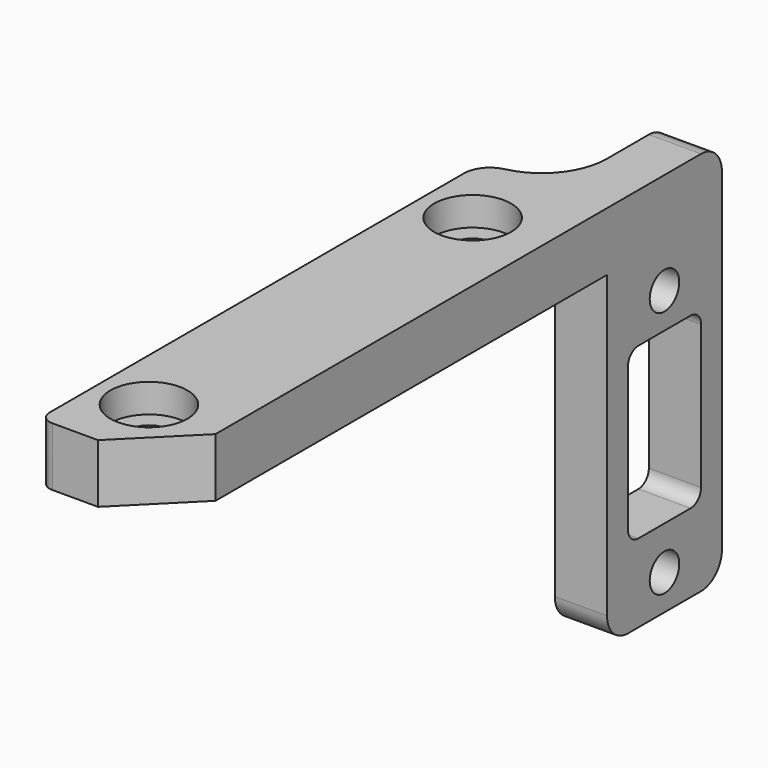
from build123d import *

# Parameters (mm, degrees)
F0_W           = 9.5
F0_H           = 42.5
F1_DEPTH       = 4.5
F3_D           = 3.1
F3_CBORE_D     = 5.9
F3_CBORE_DEPTH = 2.2
F4_W           = 11
F4_H           = 29.5
F5_DEPTH       = 4
F7_D           = 2.83
F8_W           = 7
F8_H           = 13
F9_DEPTH       = 25
F10_T1_DEPTH   = 4.5
F11_R          = 2
F12_SIZE       = 5
F13_R          = 1


# Not quite as in the source:
# - a fillet or chamfer that OpenCascade refuses, or shapes differently, is made with other operations: its cross-section is extruded or revolved along the edge and cut away or added


with BuildPart() as f1:
    # F0 (on Top) → F1 (new body)
    with BuildSketch(Plane.XY):
        with Locations((-4.75, 21.25)):
            Rectangle(F0_W, F0_H)
    extrude(amount=F1_DEPTH)

    # F3 (through all)
    with Locations(Plane.XY.offset(4.5)):
        with Locations((-5.5, 36.5), (-5.5, 5.5)):
            CounterBoreHole(F3_D / 2, F3_CBORE_D / 2, F3_CBORE_DEPTH)

    # F4 (on Right) → F5 (join)
    with BuildSketch(Plane.YZ):
        with Locations((48, -10.25)):
            Rectangle(F4_W, F4_H)
    extrude(amount=-F5_DEPTH)

    # F7 (through all)
    with Locations(Plane.YZ):
        with Locations((48, -3.3), (48, -22.3)):
            Hole(F7_D / 2)

    # F8 (on face) → F9 (cut)
    with BuildSketch(Plane.YZ):
        with Locations((48, -12.5)):
            Rectangle(F8_W, F8_H)
    extrude(amount=-F9_DEPTH, mode=Mode.SUBTRACT)

    # F10: fillet of radius 5 on 1 edges, made by hand

    # F10_s2 → F10_t1 (join)
    with BuildSketch(Plane.XY):
        with BuildLine():
            ThreePointArc((-9.0009656854, 42.4996), (-5.4644660941, 43.9644660941), (-3.9996, 47.5009656854))
            Line((-3.9996, 47.5009656854), (-3.4994634315, 47.5009656854))
            ThreePointArc((-3.4994634315, 47.5009656854), (-3.4998634315, 45.0004828427), (-3.4998634315, 42.5))
            Line((-3.4998634315, 42.5), (-4, 41.9998634315))
            ThreePointArc((-4, 41.9998634315), (-6.5004828427, 41.9998634315), (-9.0009656854, 41.9994634315))
            Line((-9.0009656854, 41.9994634315), (-9.0009656854, 42.4996))
        make_face()
    extrude(amount=F10_T1_DEPTH)

    # F11
    f11_edges = [f1.edges().sort_by_distance(p)[0] for p in [
        (-2, 53.5, 4.5),
        (-2, 53.5, -25),
        (-2, 42.5, -25),
        (-9.5, 42.5, 2.25),
    ]]
    fillet(f11_edges, radius=F11_R)

    # F12
    f12_edges = [f1.edges().sort_by_distance(p)[0] for p in [
        (0, 0, 2.25),
    ]]
    chamfer(f12_edges, length=F12_SIZE)

    # F13
    f13_edges = [f1.edges().sort_by_distance(p)[0] for p in [
        (-2, 44.5, -6),
        (-2, 51.5, -6),
        (-2, 44.5, -19),
        (-2, 51.5, -19),
        (-9.5, 0, 2.25),
    ]]
    fillet(f13_edges, radius=F13_R)


solid = f1.part
